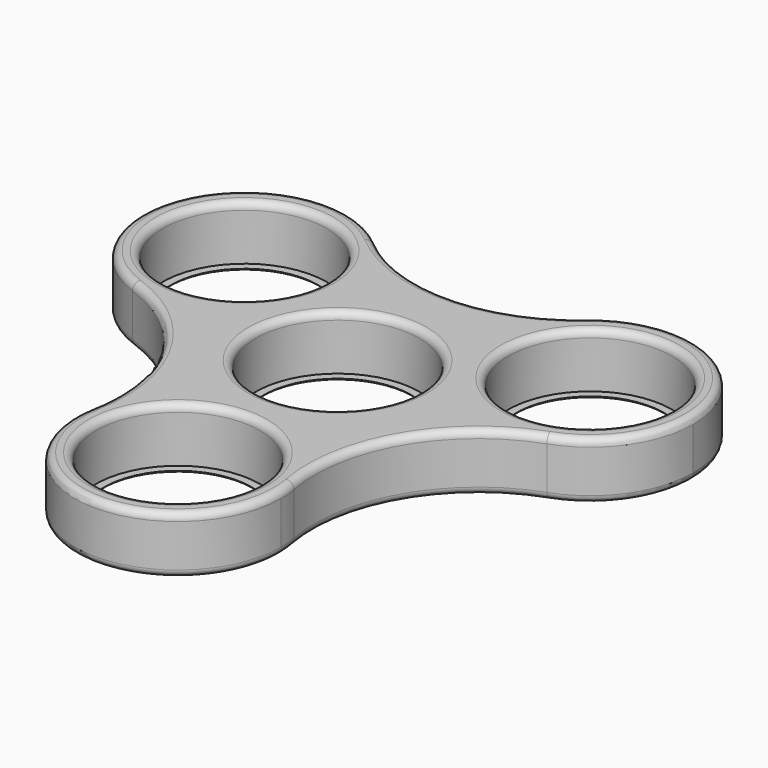
from build123d import *

# Parameters (mm, degrees)
F0_R         = 11.15
F1_DEPTH     = 7.8
F2_R         = 11.15
F2_R_2       = 10
F3_DEPTH     = 0.4
F4_R         = 11.15
F4_R_2       = 10
F5_DEPTH     = 0.4
F6_T10_ANGLE = 80.8915948213
F6_T12_ANGLE = 200.8915947618
F6_T14_ANGLE = 80.8915945525
F6_T16_ANGLE = 200.8915947547
F6_T18_ANGLE = 80.8915942666
F6_T20_ANGLE = 200.8915950895
F6_T22_ANGLE = 80.8915948213
F6_T24_ANGLE = 200.8915947618
F6_T26_ANGLE = 80.8915945525
F6_T28_ANGLE = 200.8915947547
F6_T30_ANGLE = 80.8915942666
F6_T32_ANGLE = 200.8915950895


# Not quite as in the source:
# - a fillet or chamfer that OpenCascade refuses, or shapes differently, is made with other operations: its cross-section is extruded or revolved along the edge and cut away or added


with BuildPart() as f1:
    # F0 (on Top) → F1 (new body)
    with BuildSketch(Plane.XY):
        with BuildLine():
            ThreePointArc((-14.4178023884, 24.2220115243), (-10.7887694034, 19.434980828), (-9.5, 13.567731326))
            ThreePointArc((-9.5, 13.567731326), (-15.4253761081, 2.1309289317), (-28.1857784292, 0.3751773461))
            ThreePointArc((-28.1857784292, 0.3751773461), (-17.4686665105, -7.7494316525), (-13.3996429494, -20.567731326))
            ThreePointArc((-13.3996429494, -20.567731326), (-13.4919177982, -22.5908599334), (-13.7679761122, -24.5971888737))
            ThreePointArc((-13.7679761122, -24.5971888737), (-1.54e-08, -13.1354626519), (13.7679761066, -24.5971888434))
            ThreePointArc((13.7679761066, -24.5971888434), (16.3771898334, -9.4553750199), (28.1857783538, 0.3751773193))
            ThreePointArc((28.1857783538, 0.3751773193), (11.3756443069, 6.5677313954), (14.4178023884, 24.2220115243))
            ThreePointArc((14.4178023884, 24.2220115243), (0, 18.9107499483), (-14.4178023884, 24.2220115243))
        make_face()
        Circle(F0_R, mode=Mode.SUBTRACT)
        with BuildLine():
            ThreePointArc((-28.1857784292, 0.3751773461), (-15.4253761081, 2.1309289317), (-9.5, 13.567731326))
            ThreePointArc((-9.5, 13.567731326), (-10.7887694034, 19.434980828), (-14.4178023884, 24.2220115243))
            ThreePointArc((-14.4178023884, 24.2220115243), (-35.6243556731, 20.5677312911), (-28.1857784292, 0.3751773461))
        make_face()
        with Locations((-23.5, 13.567731326)):
            Circle(F0_R, mode=Mode.SUBTRACT)
        with BuildLine():
            ThreePointArc((37.5, 13.567731326), (29.367249502, 26.2789619226), (14.4178023884, 24.2220115243))
            ThreePointArc((14.4178023884, 24.2220115243), (11.3756443069, 6.5677313954), (28.1857783538, 0.3751773193))
            ThreePointArc((28.1857783538, 0.3751773193), (34.9368023711, 5.4931074014), (37.5, 13.567731326))
        make_face()
        with Locations((23.5, 13.567731326)):
            Circle(F0_R, mode=Mode.SUBTRACT)
        with BuildLine():
            ThreePointArc((13.7679761066, -24.5971888434), (-1.54e-08, -13.1354626519), (-13.7679761122, -24.5971888737))
            ThreePointArc((-13.7679761122, -24.5971888737), (-1.2744281911, -41.0773360119), (14, -27.1354626519))
            ThreePointArc((14, -27.1354626519), (13.9418733586, -25.8610344454), (13.7679761066, -24.5971888434))
        make_face()
        with Locations((0, -27.1354626519)):
            Circle(F0_R, mode=Mode.SUBTRACT)
    extrude(amount=F1_DEPTH)

    # F2 (on face) → F3 (join)
    with BuildSketch(Plane(origin=(0, 0, 0), x_dir=(1, 0, 0), z_dir=(0, 0, -1))):
        with Locations((0, 27.1354626519)):
            Circle(F2_R)
        with Locations((0, 27.1354626519)):
            Circle(F2_R_2, mode=Mode.SUBTRACT)
        with Locations((23.5, -13.567731326)):
            Circle(F2_R)
        with Locations((23.5, -13.567731326)):
            Circle(F2_R_2, mode=Mode.SUBTRACT)
        with Locations((-23.5, -13.567731326)):
            Circle(F2_R)
        with Locations((-23.5, -13.567731326)):
            Circle(F2_R_2, mode=Mode.SUBTRACT)
    extrude(amount=-F3_DEPTH)

    # F4 (on face) → F5 (join)
    with BuildSketch(Plane(origin=(0, 0, 0), x_dir=(1, 0, 0), z_dir=(0, 0, -1))):
        Circle(F4_R)
        Circle(F4_R_2, mode=Mode.SUBTRACT)
    extrude(amount=-F5_DEPTH)

    # F6: fillet of radius 1 on 20 edges, made by hand

    # F6_s1 → F6_t2 (revolve, cut)
    with BuildSketch(Plane.XZ.offset(-13.567731326)):
        with BuildLine():
            ThreePointArc((-11.35, 7.8), (-12.0571067812, 7.5071067812), (-12.35, 6.8))
            Line((-12.35, 6.8), (-12.35, 7.8))
            Line((-12.35, 7.8), (-11.35, 7.8))
        make_face()
    revolve(axis=Axis((-23.5, 13.567731326, 7.8), (0, 0, 1)), mode=Mode.SUBTRACT)

    # F6_s3 → F6_t4 (revolve, cut)
    with BuildSketch(Plane.XZ.offset(27.1354626519)):
        with BuildLine():
            ThreePointArc((12.15, 7.8), (11.4428932188, 7.5071067812), (11.15, 6.8))
            Line((11.15, 6.8), (11.15, 7.8))
            Line((11.15, 7.8), (12.15, 7.8))
        make_face()
    revolve(axis=Axis((0, -27.1354626519, 7.8), (0, 0, 1)), mode=Mode.SUBTRACT)

    # F6_s5 → F6_t6 (revolve, cut)
    with BuildSketch(Plane.XZ):
        with BuildLine():
            ThreePointArc((12.15, 7.8), (11.4428932188, 7.5071067812), (11.15, 6.8))
            Line((11.15, 6.8), (11.15, 7.8))
            Line((11.15, 7.8), (12.15, 7.8))
        make_face()
    revolve(axis=Axis((0, 0, 7.8), (0, 0, 1)), mode=Mode.SUBTRACT)

    # F6_s7 → F6_t8 (revolve, cut)
    with BuildSketch(Plane.XZ.offset(-13.567731326)):
        with BuildLine():
            ThreePointArc((35.65, 7.8), (34.9428932188, 7.5071067812), (34.65, 6.8))
            Line((34.65, 6.8), (34.65, 7.8))
            Line((34.65, 7.8), (35.65, 7.8))
        make_face()
    revolve(axis=Axis((23.5, 13.567731326, 7.8), (0, 0, 1)), mode=Mode.SUBTRACT)

    # F6_s9 → F6_t10 (revolve, cut)
    with BuildSketch(Plane(origin=(20.3083844645, 17.3117994564, 0), x_dir=(0, 0, 1), z_dir=(0.761020012, 0.6487284034, 0))):
        with BuildLine():
            ThreePointArc((6.8, -9.0801975759), (7.5071067812, -8.7873043571), (7.8, -8.0801975759))
            Line((7.8, -8.0801975759), (7.8, -9.0801975759))
            Line((7.8, -9.0801975759), (6.8, -9.0801975759))
        make_face()
    revolve(axis=Axis((0, 41.1354626519, 7.8), (0, 0, -1)), revolution_arc=F6_T10_ANGLE, mode=Mode.SUBTRACT)

    # F6_s11 → F6_t12 (revolve, cut)
    with BuildSketch(Plane(origin=(-20.3083844997, 17.3117993675, 0), x_dir=(0, 0, 1), z_dir=(0.7610200142, -0.6487284008, 0))):
        with BuildLine():
            ThreePointArc((6.8, -9.0801976664), (7.5071067812, -8.7873044476), (7.8, -8.0801976664))
            Line((7.8, -8.0801976664), (7.8, -9.0801976664))
            Line((7.8, -9.0801976664), (6.8, -9.0801976664))
        make_face()
    revolve(axis=Axis((-23.5, 13.567731326, 7.8), (0, 0, 1)), revolution_arc=F6_T12_ANGLE, mode=Mode.SUBTRACT)

    # F6_s13 → F6_t14 (revolve, cut)
    with BuildSketch(Plane(origin=(-25.1466502077, 8.9316771809, 0), x_dir=(0, 0, 1), z_dir=(-0.9423252823, 0.3346984649, 0))):
        with BuildLine():
            ThreePointArc((7.8, -8.0801976725), (7.5071067812, -8.7873044537), (6.8, -9.0801976725))
            Line((6.8, -9.0801976725), (7.8, -9.0801976725))
            Line((7.8, -9.0801976725), (7.8, -8.0801976725))
        make_face()
    revolve(axis=Axis((-35.624355653, -20.567731326, 7.8), (0, 0, -1)), revolution_arc=F6_T14_ANGLE, mode=Mode.SUBTRACT)

    # F6_s15 → F6_t16 (revolve, cut)
    with BuildSketch(Plane(origin=(-4.8382658309, -26.2434765539, 0), x_dir=(0, 0, 1), z_dir=(0.1813052699, 0.9834268652, 0))):
        with BuildLine():
            ThreePointArc((7.8, -8.0801976209), (7.5071067812, -8.787304402), (6.8, -9.0801976209))
            Line((6.8, -9.0801976209), (7.8, -9.0801976209))
            Line((7.8, -9.0801976209), (7.8, -8.0801976209))
        make_face()
    revolve(axis=Axis((0, -27.1354626519, 7.8), (0, 0, 1)), revolution_arc=F6_T16_ANGLE, mode=Mode.SUBTRACT)

    # F6_s17 → F6_t18 (revolve, cut)
    with BuildSketch(Plane(origin=(4.8382658036, -26.2434765203, 0), x_dir=(0, 0, 1), z_dir=(0.1813052691, -0.9834268653, 0))):
        with BuildLine():
            ThreePointArc((7.8, -8.0801976417), (7.5071067812, -8.7873044229), (6.8, -9.0801976417))
            Line((6.8, -9.0801976417), (7.8, -9.0801976417))
            Line((7.8, -9.0801976417), (7.8, -8.0801976417))
        make_face()
    revolve(axis=Axis((35.624355653, -20.567731326, 7.8), (0, 0, -1)), revolution_arc=F6_T18_ANGLE, mode=Mode.SUBTRACT)

    # F6_s19 → F6_t20 (revolve, cut)
    with BuildSketch(Plane(origin=(25.1466503366, 8.9316768958, 0), x_dir=(0, 0, 1), z_dir=(-0.9423252862, -0.3346984538, 0))):
        with BuildLine():
            ThreePointArc((6.8, -9.0801973606), (7.5071067812, -8.7873041418), (7.8, -8.0801973606))
            Line((7.8, -8.0801973606), (7.8, -9.0801973606))
            Line((7.8, -9.0801973606), (6.8, -9.0801973606))
        make_face()
    revolve(axis=Axis((23.5, 13.567731326, 7.8), (0, 0, 1)), revolution_arc=F6_T20_ANGLE, mode=Mode.SUBTRACT)

    # F6_s21 → F6_t22 (revolve, cut)
    with BuildSketch(Plane(origin=(20.3083844645, 17.3117994564, 0), x_dir=(0, 0, 1), z_dir=(0.761020012, 0.6487284034, 0))):
        with BuildLine():
            ThreePointArc((1, -9.0801975759), (0.2928932188, -8.7873043571), (0, -8.0801975759))
            Line((0, -8.0801975759), (0, -9.0801975759))
            Line((0, -9.0801975759), (1, -9.0801975759))
        make_face()
    revolve(axis=Axis((0, 41.1354626519, 0), (0, 0, -1)), revolution_arc=F6_T22_ANGLE, mode=Mode.SUBTRACT)

    # F6_s23 → F6_t24 (revolve, cut)
    with BuildSketch(Plane(origin=(-20.3083844997, 17.3117993675, 0), x_dir=(0, 0, 1), z_dir=(0.7610200142, -0.6487284008, 0))):
        with BuildLine():
            ThreePointArc((1, -9.0801976664), (0.2928932188, -8.7873044476), (0, -8.0801976664))
            Line((0, -8.0801976664), (0, -9.0801976664))
            Line((0, -9.0801976664), (1, -9.0801976664))
        make_face()
    revolve(axis=Axis((-23.5, 13.567731326, 0), (0, 0, 1)), revolution_arc=F6_T24_ANGLE, mode=Mode.SUBTRACT)

    # F6_s25 → F6_t26 (revolve, cut)
    with BuildSketch(Plane(origin=(-25.1466502077, 8.9316771809, 0), x_dir=(0, 0, 1), z_dir=(-0.9423252823, 0.3346984649, 0))):
        with BuildLine():
            ThreePointArc((0, -8.0801976725), (0.2928932188, -8.7873044537), (1, -9.0801976725))
            Line((1, -9.0801976725), (0, -9.0801976725))
            Line((0, -9.0801976725), (0, -8.0801976725))
        make_face()
    revolve(axis=Axis((-35.624355653, -20.567731326, 0), (0, 0, -1)), revolution_arc=F6_T26_ANGLE, mode=Mode.SUBTRACT)

    # F6_s27 → F6_t28 (revolve, cut)
    with BuildSketch(Plane(origin=(-4.8382658309, -26.2434765539, 0), x_dir=(0, 0, 1), z_dir=(0.1813052699, 0.9834268652, 0))):
        with BuildLine():
            ThreePointArc((0, -8.0801976209), (0.2928932188, -8.787304402), (1, -9.0801976209))
            Line((1, -9.0801976209), (0, -9.0801976209))
            Line((0, -9.0801976209), (0, -8.0801976209))
        make_face()
    revolve(axis=Axis((0, -27.1354626519, 0), (0, 0, 1)), revolution_arc=F6_T28_ANGLE, mode=Mode.SUBTRACT)

    # F6_s29 → F6_t30 (revolve, cut)
    with BuildSketch(Plane(origin=(4.8382658036, -26.2434765203, 0), x_dir=(0, 0, 1), z_dir=(0.1813052691, -0.9834268653, 0))):
        with BuildLine():
            ThreePointArc((0, -8.0801976417), (0.2928932188, -8.7873044229), (1, -9.0801976417))
            Line((1, -9.0801976417), (0, -9.0801976417))
            Line((0, -9.0801976417), (0, -8.0801976417))
        make_face()
    revolve(axis=Axis((35.624355653, -20.567731326, 0), (0, 0, -1)), revolution_arc=F6_T30_ANGLE, mode=Mode.SUBTRACT)

    # F6_s31 → F6_t32 (revolve, cut)
    with BuildSketch(Plane(origin=(25.1466503366, 8.9316768958, 0), x_dir=(0, 0, 1), z_dir=(-0.9423252862, -0.3346984538, 0))):
        with BuildLine():
            ThreePointArc((1, -9.0801973606), (0.2928932188, -8.7873041418), (0, -8.0801973606))
            Line((0, -8.0801973606), (0, -9.0801973606))
            Line((0, -9.0801973606), (1, -9.0801973606))
        make_face()
    revolve(axis=Axis((23.5, 13.567731326, 0), (0, 0, 1)), revolution_arc=F6_T32_ANGLE, mode=Mode.SUBTRACT)

    # F6_s33 → F6_t34 (revolve, cut)
    with BuildSketch(Plane.XZ.offset(-13.567731326)):
        with BuildLine():
            ThreePointArc((-12.7, 0), (-13.1472135955, 0.105572809), (-13.5, 0.4))
            Line((-13.5, 0.4), (-13.5, 0))
            Line((-13.5, 0), (-12.7, 0))
        make_face()
    revolve(axis=Axis((-23.5, 13.567731326, 0), (0, 0, -1)), mode=Mode.SUBTRACT)

    # F6_s35 → F6_t36 (revolve, cut)
    with BuildSketch(Plane.XZ.offset(-13.567731326)):
        with BuildLine():
            ThreePointArc((34.3, 0), (33.8527864045, 0.105572809), (33.5, 0.4))
            Line((33.5, 0.4), (33.5, 0))
            Line((33.5, 0), (34.3, 0))
        make_face()
    revolve(axis=Axis((23.5, 13.567731326, 0), (0, 0, -1)), mode=Mode.SUBTRACT)

    # F6_s37 → F6_t38 (revolve, cut)
    with BuildSketch(Plane.XZ.offset(27.1354626519)):
        with BuildLine():
            ThreePointArc((10.8, 0), (10.3527864045, 0.105572809), (10, 0.4))
            Line((10, 0.4), (10, 0))
            Line((10, 0), (10.8, 0))
        make_face()
    revolve(axis=Axis((0, -27.1354626519, 0), (0, 0, -1)), mode=Mode.SUBTRACT)

    # F6_s39 → F6_t40 (revolve, cut)
    with BuildSketch(Plane.XZ):
        with BuildLine():
            ThreePointArc((10.8, 0), (10.3527864045, 0.105572809), (10, 0.4))
            Line((10, 0.4), (10, 0))
            Line((10, 0), (10.8, 0))
        make_face()
    revolve(axis=Axis((0, 0, 0), (0, 0, -1)), mode=Mode.SUBTRACT)


solid = f1.part
